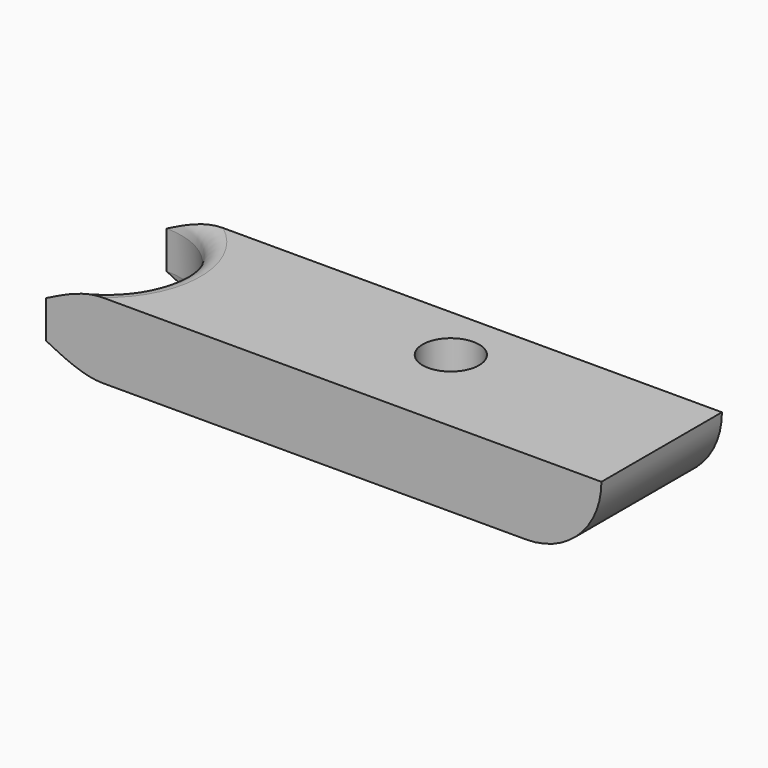
from build123d import *

# Parameters (mm, degrees)
F0_R        = 1.5
F1_DEPTH    = 4
F2_T2_ANGLE = 301.9493341655
F2_T4_ANGLE = 301.9493341655
F3_R        = 3.99999


# Not quite as in the source:
# - a fillet or chamfer that OpenCascade refuses, or shapes differently, is made with other operations: its cross-section is extruded or revolved along the edge and cut away or added
# - a fillet or chamfer is up to 0.001 mm smaller than in the source, because OpenCascade refuses the exact size


with BuildPart() as f1:
    # F0 (on Top) → F1 (new body)
    with BuildSketch(Plane.XY):
        with BuildLine():
            ThreePointArc((0, 8), (2.8284271247, 6.8284271247), (4, 4))
            ThreePointArc((4, 4), (2.8284271247, 1.1715728753), (0, 0))
            Line((0, 0), (29.5, 0))
            Line((29.5, 0), (29.5, 8))
            Line((29.5, 8), (0, 8))
        make_face()
        with Locations((17.5, 5)):
            Circle(F0_R, mode=Mode.SUBTRACT)
    extrude(amount=F1_DEPTH)

    # F2: fillet of radius 1 on 2 edges, made by hand

    # F2_s1 → F2_t2 (revolve, cut)
    with BuildSketch(Plane(origin=(1.697032729, 3.0583382808, 0), x_dir=(0, 0, 1), z_dir=(-0.4851962797, -0.8744052666, 0))):
        with BuildLine():
            ThreePointArc((1, 5.9407851187), (0.2928932188, 6.2336783375), (0, 6.9407851187))
            Line((0, 6.9407851187), (0, 5.9407851187))
            Line((0, 5.9407851187), (1, 5.9407851187))
        make_face()
    revolve(axis=Axis((0, 4, 0), (0, 0, -1)), revolution_arc=F2_T2_ANGLE, mode=Mode.SUBTRACT)

    # F2_s3 → F2_t4 (revolve, cut)
    with BuildSketch(Plane(origin=(-1.697032729, 3.0583382808, 0), x_dir=(0, 0, 1), z_dir=(-0.4851962797, 0.8744052666, 0))):
        with BuildLine():
            ThreePointArc((3, -2.0592148813), (3.7071067812, -2.3521081002), (4, -3.0592148813))
            Line((4, -3.0592148813), (4, -2.0592148813))
            Line((4, -2.0592148813), (3, -2.0592148813))
        make_face()
    revolve(axis=Axis((0, 4, 4), (0, 0, 1)), revolution_arc=F2_T4_ANGLE, mode=Mode.SUBTRACT)

    # F3 (radius 4 in the source; OpenCascade refuses exactly that, so slightly less here)
    f3_edges = [f1.edges().sort_by_distance(p)[0] for p in [
        (29.5, 4, 0),
    ]]
    fillet(f3_edges, radius=F3_R)


solid = f1.part
